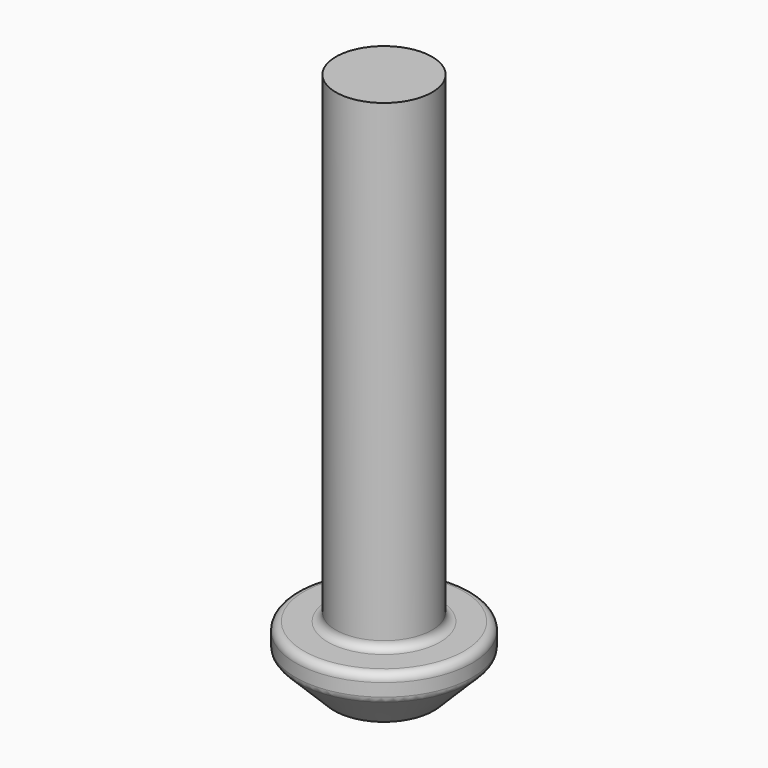
from build123d import *

# Parameters (mm, degrees)
F1_R     = 2.75
F1_R_2   = 1.5
F2_DEPTH = 2
F3_START = 1.5
F3_DEPTH = 0.5
F4_START = 2
F4_DEPTH = 15
F5_SIZE2 = 1.25
F5_SIZE  = 1.25
F6_R     = 0.25


# Not quite as in the source:
# - a feature names something its author has since deleted; it is built from what else it names


with BuildPart() as f2:
    # F1 (on Top) → F2 (new body)
    with BuildSketch(Plane.XY):
        Circle(F1_R)
        Circle(F1_R_2, mode=Mode.SUBTRACT)
        Circle(F1_R_2)
        Polygon((-0.5773502692, -1), (-1.1547005384, 0), (-0.5773502692, 1), (0.5773502692, 1), (1.1547005384, 0), (0.5773502692, -1), align=None, mode=Mode.SUBTRACT)
    extrude(amount=F2_DEPTH)

    # F1 (on Top) → F3 (join)
    with BuildSketch(Plane.XY.offset(F3_START)):
        Polygon((-0.5773502692, 1), (-1.1547005384, 0), (-0.5773502692, -1), (0.5773502692, -1), (1.1547005384, 0), (0.5773502692, 1), align=None)
    extrude(amount=F3_DEPTH)

    # F1 (on Top) → F4 (join)
    with BuildSketch(Plane.XY.offset(F4_START)):
        Circle(F1_R_2)
        Polygon((-0.5773502692, -1), (-1.1547005384, 0), (-0.5773502692, 1), (0.5773502692, 1), (1.1547005384, 0), (0.5773502692, -1), align=None, mode=Mode.SUBTRACT)
        Polygon((-0.5773502692, 1), (-1.1547005384, 0), (-0.5773502692, -1), (0.5773502692, -1), (1.1547005384, 0), (0.5773502692, 1), align=None)
    extrude(amount=F4_DEPTH)

    # F5
    f5_edges = [f2.edges().sort_by_distance(p)[0] for p in [
        (-2.75, 0, 0),
    ]]
    chamfer(f5_edges, length=F5_SIZE, length2=F5_SIZE2)

    # F6
    f6_edges = [f2.edges().sort_by_distance(p)[0] for p in [
        (-2.75, 0, 2),
        (-1.5, 0, 2),
        (-1.5, 0, 0),
        (-2.75, 0, 1.25),
    ]]
    fillet(f6_edges, radius=F6_R)


solid = f2.part
